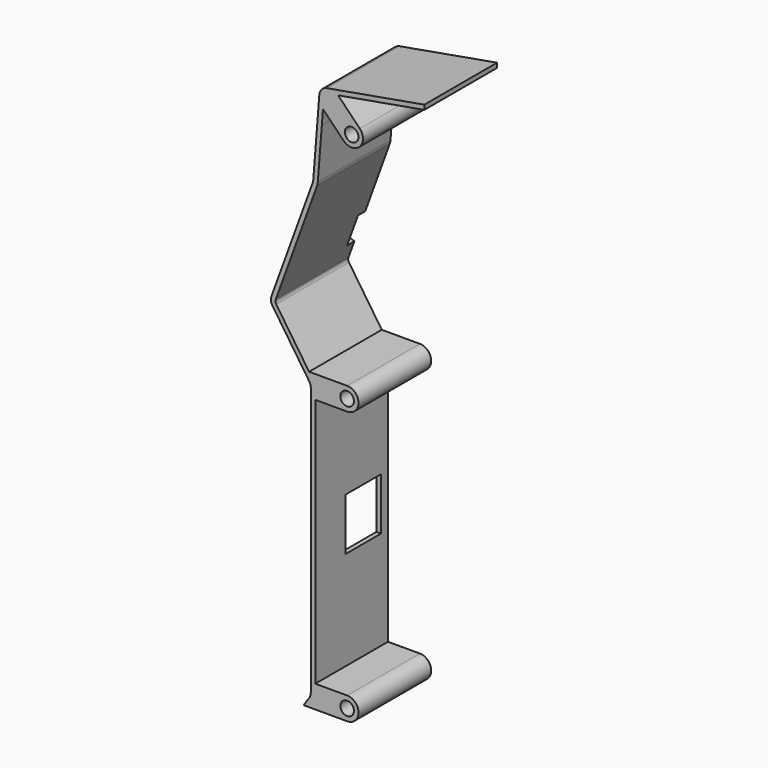
from build123d import *

# Parameters (mm, degrees)
F1_R     = 1.5
F2_DEPTH = 20
F3_W     = 2
F3_H     = 7
F4_DEPTH = 25
F5_W     = 9.7
F5_H     = 11.5
F6_DEPTH = 25


# Not quite as in the source:
# - ends of sketch curves that miss each other by under 0.0002 mm in the source are joined


with BuildPart() as f2:
    # F1 (on Front) → F2 (new body)
    with BuildSketch(Plane.XZ):
        with BuildLine():
            Line((-22.3164947392, 83.8837339027), (-17.7874447277, 79.2521323433))
            ThreePointArc((-17.7874447277, 79.2521323433), (-14.2521323433, 79.2125552723), (-14.2125552723, 82.7478676567))
            Line((-14.2125552723, 82.7478676567), (-18.9921983086, 87.6357364337))
            Line((-18.9921983086, 87.6357364337), (-17.5868240881, 87.8835418245))
            Line((-17.5868240881, 87.8835418245), (-14.5868240881, 88.4125227619))
            Line((-14.5868240881, 88.4125227619), (0, 90.9845733884))
            Line((0, 90.9845733884), (0, 92))
            Line((0, 92), (-21.474961, 88.213385))
            ThreePointArc((-21.474961, 88.213385), (-22.6081005709, 87.5885032671), (-23.1214986845, 86.4006879752))
            Line((-23.1214986845, 86.4006879752), (-24.456969, 69.431938))
            ThreePointArc((-24.456969, 69.431938), (-24.4963407526, 69.1645008146), (-24.5714176946, 68.9048158888))
            Line((-24.5714176946, 68.9048158888), (-33.651464, 43.957595))
            ThreePointArc((-33.651464, 43.957595), (-33.757171385, 43.0298159786), (-33.4301544738, 42.1551686804))
            Line((-33.4301544738, 42.1551686804), (-25.341925, 30.163876))
            ThreePointArc((-25.341925, 30.163876), (-25.0873905233, 29.6302335248), (-25, 29.04549))
            Line((-25, 29.04549), (-25, 27))
            Line((-25, 27), (-25, -0.5))
            Line((-25, -0.5), (-24.0000002534, -0.5))
            Line((-24.0000002534, -0.5), (-24.0000002534, 27))
            Line((-24.0000002534, 27), (-17, 27))
            ThreePointArc((-17, 27), (-14.5, 29.5), (-17, 32))
            Line((-17, 32), (-25, 32))
            Line((-25, 32), (-25.3741885909, 32))
            Line((-25.3741885909, 32), (-32.6011163068, 42.7143612935))
            ThreePointArc((-32.6011163068, 42.7143612935), (-32.7646248248, 43.1516847064), (-32.7117713086, 43.6155740346))
            Line((-32.7117713086, 43.6155740346), (-23.6317251212, 68.5627955495))
            ThreePointArc((-23.6317251212, 68.5627955495), (-23.5191096678, 68.9523229367), (-23.4600509821, 69.3534786388))
            Line((-23.4600509821, 69.3534786388), (-22.5711850089, 80.6475881907))
            Line((-22.5711850089, 80.6475881907), (-22.3164947392, 83.8837339027))
        make_face()
        with Locations((-17, 29.5)):
            Circle(F1_R, mode=Mode.SUBTRACT)
        with Locations((-16, 81)):
            Circle(F1_R, mode=Mode.SUBTRACT)
        with BuildLine():
            Line((-24.0000002534, -28), (-24.0000002534, -0.5))
            Line((-24.0000002534, -0.5), (-25, -0.5))
            Line((-25, -0.5), (-25, -30.04549))
            ThreePointArc((-25, -30.04549), (-25.0873905233, -30.6302335248), (-25.3419249898, -31.1638760069))
            Line((-25.341925, -31.163876), (-26.5804062367, -33))
            Line((-26.5804062367, -33), (-25, -33))
            Line((-25, -33), (-17, -33))
            ThreePointArc((-17, -33), (-14.5, -30.5), (-17, -28))
            Line((-17, -28), (-24.0000002534, -28))
        make_face()
        with Locations((-17, -30.5)):
            Circle(F1_R, mode=Mode.SUBTRACT)
    extrude(amount=F2_DEPTH)

    # F3 (on face) → F4 (cut)
    with BuildSketch(Plane(origin=(-43.8426892635, 0, 15.9574341077), x_dir=(0, -1, 0), z_dir=(-0.9396926192, 0, 0.3420201476))):
        with Locations((1, 37.1150750518)):
            Rectangle(F3_W, F3_H)
    extrude(amount=-F4_DEPTH, mode=Mode.SUBTRACT)

    # F5 (on face) → F6 (cut)
    with BuildSketch(Plane(origin=(-25, 0, 0), x_dir=(0, -1, 0), z_dir=(-1, 0, 0))):
        with Locations((6.8, -0.5)):
            Rectangle(F5_W, F5_H)
    extrude(amount=-F6_DEPTH, mode=Mode.SUBTRACT)


solid = f2.part
